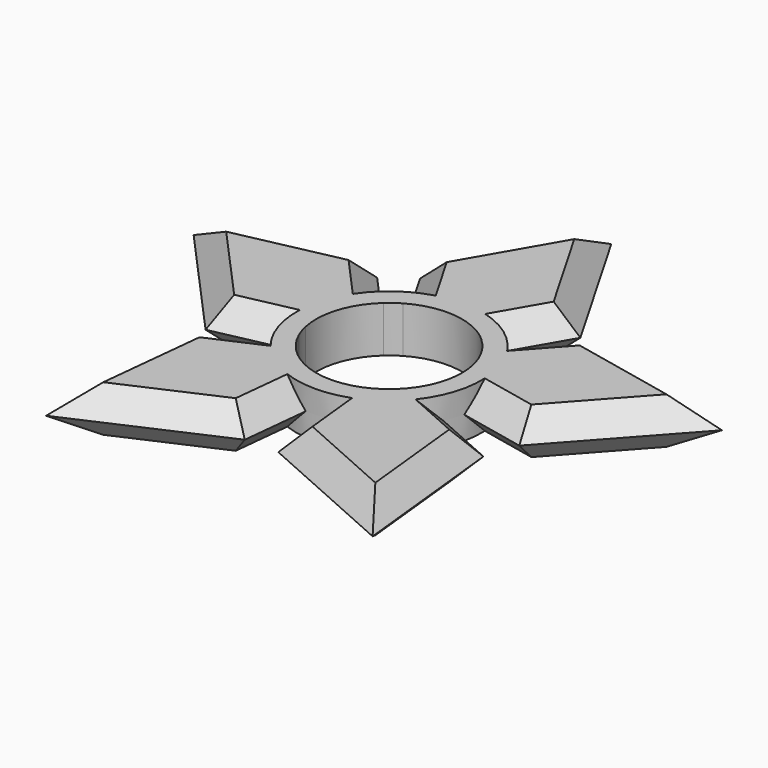
from build123d import *

# Parameters (mm, degrees)
F1_DEPTH = 7
F2_COUNT = 5
F3_SIZE  = 3.49999


# Not quite as in the source:
# - a fillet or chamfer is up to 0.001 mm smaller than in the source, because OpenCascade refuses the exact size


with BuildPart() as f1:
    # F0 (on Top) → F1 (new body)
    with BuildSketch(Plane.XY):
        Polygon((-12.124355653, 11.8902331595), (12.124355653, 11.8902331595), (0, 32.8902331595), align=None)
        with BuildLine():
            Line((7, 3.0145888124), (12.124355653, 11.8902331595))
            Line((12.124355653, 11.8902331595), (-12.124355653, 11.8902331595))
            Line((-12.124355653, 11.8902331595), (-7, 3.0145888124))
            ThreePointArc((-7, 3.0145888124), (0, 4.8902331595), (7, 3.0145888124))
        make_face()
        with BuildLine():
            Line((5.5125, 0.4381632362), (7, 3.0145888124))
            ThreePointArc((7, 3.0145888124), (0, 4.8902331595), (-7, 3.0145888124))
            Line((-7, 3.0145888124), (-5.5125, 0.4381632362))
            ThreePointArc((-5.5125, 0.4381632362), (0, 1.9152331595), (5.5125, 0.4381632362))
        make_face()
        with BuildLine():
            ThreePointArc((14, -9.1097668405), (12.124355653, -2.1097668405), (7, 3.0145888124))
            Line((7, 3.0145888124), (5.5125, 0.4381632362))
            ThreePointArc((5.5125, 0.4381632362), (9.5479300767, -3.5972668405), (11.025, -9.1097668405))
            ThreePointArc((11.025, -9.1097668405), (-5.5125, -18.6576969173), (-5.5125, 0.4381632362))
            Line((-5.5125, 0.4381632362), (-7, 3.0145888124))
            ThreePointArc((-7, 3.0145888124), (-7, -21.2341224935), (14, -9.1097668405))
        make_face()
    extrude(amount=F1_DEPTH)

    # F2: F1 ×5 about axis
    f2_axis = Axis((0, -9.1097668405, 0), (0, 0, -1))


with BuildPart() as f1_1:
    add(f1.part)
    for i in range(1, F2_COUNT):
        add(f1.part.rotate(f2_axis, i * 360 / F2_COUNT))

    # F3 (size 3.5 in the source; OpenCascade refuses exactly that, so slightly less here)
    f3_edges = [f1_1.edges().sort_by_distance(p)[0] for p in [
        (-13.610831, -38.157061, 7),
        (-23.41964, -31.030543, 7),
        (-18.706443, -13.085944, 7),
        (-17.470968, -16.888343, 7),
        (-31.831596, -5.141205, 7),
        (-28.084964, 6.389742, 7),
        (-9.562178, 7.452411, 7),
        (-12.796692, 5.102399, 7),
        (-6.062178, 22.390233, 7),
        (6.062178, 22.390233, 7),
        (9.562178, 7.452411, 7),
        (12.796692, 5.102399, 7),
        (28.084964, 6.389742, 7),
        (31.831596, -5.141205, 7),
        (18.706443, -13.085944, 7),
        (17.470968, -16.888343, 7),
        (23.41964, -31.030543, 7),
        (13.610831, -38.157061, 7),
        (1.99904, -28.129357, 7),
        (-1.99904, -28.129357, 7),
        (-13.610831, -38.157061, 0),
        (-23.41964, -31.030543, 0),
        (-1.99904, -28.129357, 0),
        (1.99904, -28.129357, 0),
        (13.610831, -38.157061, 0),
        (23.41964, -31.030543, 0),
        (17.470968, -16.888343, 0),
        (18.706443, -13.085944, 0),
        (31.831596, -5.141205, 0),
        (28.084964, 6.389742, 0),
        (12.796692, 5.102399, 0),
        (9.562178, 7.452411, 0),
        (6.062178, 22.390233, 0),
        (-6.062178, 22.390233, 0),
        (-9.562178, 7.452411, 0),
        (-12.796692, 5.102399, 0),
        (-28.084964, 6.389742, 0),
        (-31.831596, -5.141205, 0),
        (-18.706443, -13.085944, 0),
        (-17.470968, -16.888343, 0),
    ]]
    chamfer(f3_edges, length=F3_SIZE)


solid = f1_1.part
